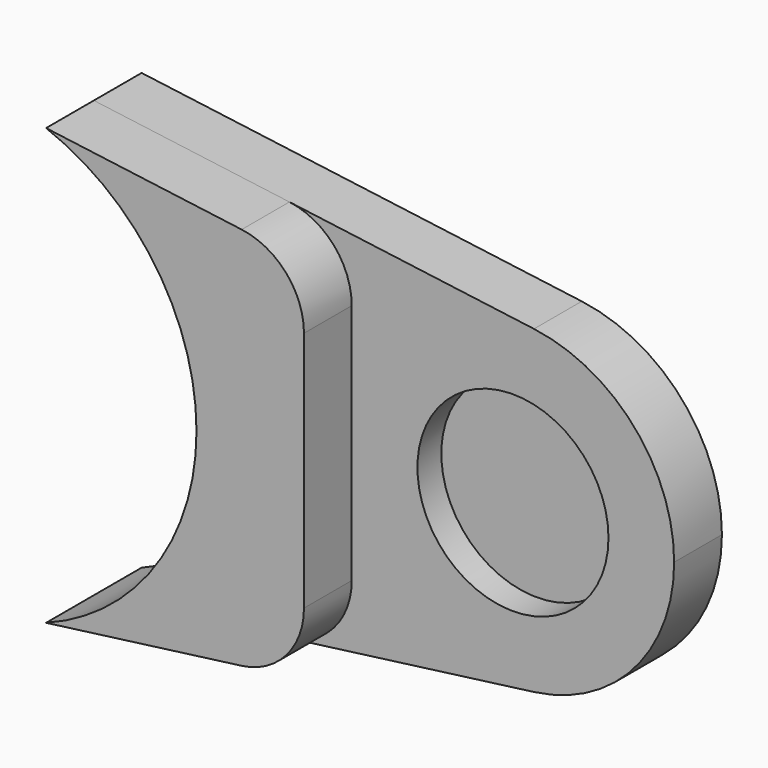
from build123d import *

# Parameters (mm, degrees)
F0_R         = 8
F1_DEPTH     = 10
F2_R         = 1.5
F3_DEPTH     = 22.1
F4_R         = 1.4
F5_DEPTH     = 8
F6_T1_DEPTH  = 25.4217528018
F7_R         = 2
F8_R         = 2
F10_DEPTH    = 2.5
F11_R        = 4
F12_DEPTH    = 6
F14_DEPTH    = 2.5
F15_T1_DEPTH = 9.0773234724
F17_DEPTH    = 25
F18_DEPTH    = 7.25


# Not quite as in the source:
# - a fillet or chamfer that OpenCascade refuses, or shapes differently, is made with other operations: its cross-section is extruded or revolved along the edge and cut away or added


with BuildPart() as f1:
    # F0 (on Front) → F1 (new body)
    with BuildSketch(Plane.XZ):
        with BuildLine():
            ThreePointArc((-5.123475383, -8), (4.5594398703, -8.3343570879), (9.5, 0))
            ThreePointArc((9.5, 0), (2.5991730895, 9.1375215048), (-8.0777472107, 5))
            ThreePointArc((-8.0777472107, 5), (-8.4879541617, 4.2666888975), (-8.8317608663, 3.5))
            ThreePointArc((-8.8317608663, 3.5), (-9.0415515645, -2.9155351664), (-5.123475383, -8))
        make_face()
        Circle(F0_R, mode=Mode.SUBTRACT)
        with BuildLine():
            ThreePointArc((-8.8317608663, 3.5), (-8.4879541617, 4.2666888975), (-8.0777472107, 5))
            Line((-8.0777472107, 5), (-23.5, 5))
            ThreePointArc((-23.5, 5), (-24.7247448714, 4.5811388301), (-25.4364916731, 3.5))
            Line((-25.4364916731, 3.5), (-8.8317608663, 3.5))
        make_face()
        with BuildLine():
            Line((-23.5, -8), (-5.123475383, -8))
            ThreePointArc((-5.123475383, -8), (-9.0415515645, -2.9155351664), (-8.8317608663, 3.5))
            Line((-8.8317608663, 3.5), (-25.4364916731, 3.5))
            ThreePointArc((-25.4364916731, 3.5), (-25.4840593925, 3.252008585), (-25.5, 3))
            Line((-25.5, 3), (-25.5, 0))
            Line((-25.5, 0), (-25.5, -3.5))
            Line((-25.5, -3.5), (-25.5, -6))
            ThreePointArc((-25.5, -6), (-24.9142135624, -7.4142135624), (-23.5, -8))
        make_face()
        with BuildLine():
            ThreePointArc((-25.5, 3), (-25.4840593925, 3.252008585), (-25.4364916731, 3.5))
            Line((-25.4364916731, 3.5), (-25.5, 3.5))
            Line((-25.5, 3.5), (-31.5, 3.5))
            ThreePointArc((-31.5, 3.5), (-32.2071067812, 3.2071067812), (-32.5, 2.5))
            Line((-32.5, 2.5), (-32.5, 1.5))
            Line((-32.5, 1.5), (-32.5, 0))
            Line((-32.5, 0), (-32.5, -1.5))
            Line((-32.5, -1.5), (-32.5, -2.5))
            ThreePointArc((-32.5, -2.5), (-32.2071067812, -3.2071067812), (-31.5, -3.5))
            Line((-31.5, -3.5), (-25.5, -3.5))
            Line((-25.5, -3.5), (-25.5, 0))
            Line((-25.5, 0), (-25.5, 3))
        make_face()
    extrude(amount=F1_DEPTH)

    # F2 (on face) → F3 (cut)
    with BuildSketch(Plane(origin=(-32.5, 0, 0), x_dir=(0, -1, 0), z_dir=(-1, 0, 0))):
        with Locations((5, 0)):
            Circle(F2_R)
    extrude(amount=-F3_DEPTH, mode=Mode.SUBTRACT)

    # F4 (on face) → F5 (cut)
    with BuildSketch(Plane(origin=(0, 0, -8), x_dir=(1, 0, 0), z_dir=(0, 0, -1))):
        with Locations((-12.4, 5)):
            Circle(F4_R)
        with Locations((-19.5, 5)):
            Circle(F4_R)
    extrude(amount=-F5_DEPTH, mode=Mode.SUBTRACT)

    # F6: fillet of radius 2 on 2 edges, made by hand

    # F6_s2 → F6_t1 (cut)
    with BuildSketch(Plane.YZ.offset(-28.4997500063)):
        with BuildLine():
            ThreePointArc((-8.0001, 5.0001), (-9.4143135624, 4.4143135624), (-10.0001, 3.0001))
            Line((-10.0001, 3.0001), (-10.0401, 3.0001))
            ThreePointArc((-10.0401, 3.0001), (-10.04, 4.00005), (-10.04, 5))
            Line((-10.04, 5), (-10, 5.04))
            ThreePointArc((-10, 5.04), (-9.00005, 5.04), (-8.0001, 5.0401))
            Line((-8.0001, 5.0401), (-8.0001, 5.0001))
        make_face()
        with BuildLine():
            ThreePointArc((-1.9999, 5.0001), (-0.5856864376, 4.4143135624), (0.0001, 3.0001))
            Line((0.0001, 3.0001), (0.0401, 3.0001))
            ThreePointArc((0.0401, 3.0001), (0.04, 4.00005), (0.04, 5))
            Line((0.04, 5), (0, 5.04))
            ThreePointArc((0, 5.04), (-0.99995, 5.04), (-1.9999, 5.0401))
            Line((-1.9999, 5.0401), (-1.9999, 5.0001))
        make_face()
    extrude(amount=F6_T1_DEPTH, mode=Mode.SUBTRACT)

    # F7
    f7_edges = [f1.edges().sort_by_distance(p)[0] for p in [
        (-32.5, -10, 0),
        (-32.5, 0, 0),
    ]]
    fillet(f7_edges, radius=F7_R)

    # F8
    f8_edges = [f1.edges().sort_by_distance(p)[0] for p in [
        (-14.311738, -10, -8),
        (-14.311738, 0, -8),
    ]]
    fillet(f8_edges, radius=F8_R)

    # F9 (on Front) → F10 (join)
    with BuildSketch(Plane.XZ):
        with BuildLine():
            ThreePointArc((0.8300844627, 8.6718317984), (6.4467419184, 5.8591147448), (8.7114698505, 0))
            Line((8.7114698505, 0), (14.25, 0))
            ThreePointArc((14.25, 0), (16.5494157481, 5.0749187005), (21.8810517975, 6.6922528143))
            Line((21.8810517975, 6.6922528143), (1.6475767802, 9.3560403352))
            Line((1.6475767802, 9.3560403352), (0.8300844627, 9.4636652405))
            Line((0.8300844627, 9.4636652405), (0.8300844627, 8.6718317984))
        make_face()
        with BuildLine():
            Line((14.25, 0), (8.7114698505, 0))
            ThreePointArc((8.7114698505, 0), (6.4467419184, -5.8591147448), (0.8300844627, -8.6718317984))
            Line((0.8300844627, -8.6718317984), (0.8300844627, -9.4636652405))
            Line((0.8300844627, -9.4636652405), (1.6475767802, -9.3560403352))
            Line((1.6475767802, -9.3560403352), (21.8810517975, -6.6922528143))
            ThreePointArc((21.8810517975, -6.6922528143), (16.5494157481, -5.0749187005), (14.25, 0))
        make_face()
        with BuildLine():
            ThreePointArc((21.8810517975, 6.6922528143), (16.5494157481, 5.0749187005), (14.25, 0))
            Line((14.25, 0), (21, 0))
            Line((21, 0), (21.8810517975, -6.6922528143))
            ThreePointArc((21.8810517975, -6.6922528143), (26.0749187005, -4.4505842519), (27.75, 0))
            ThreePointArc((27.75, 0), (26.0749187005, 4.4505842519), (21.8810517975, 6.6922528143))
        make_face()
        with BuildLine():
            Line((21, 0), (14.25, 0))
            ThreePointArc((14.25, 0), (16.5494157481, -5.0749187005), (21.8810517975, -6.6922528143))
            Line((21.8810517975, -6.6922528143), (21, 0))
        make_face()
        with BuildLine():
            Line((1.6475767802, -9.3560403352), (0.8300844627, -9.4636652405))
            ThreePointArc((0.8300844627, -9.4636652405), (1.2399988261, -9.4187261831), (1.6475767802, -9.3560403352))
        make_face()
        with BuildLine():
            ThreePointArc((1.6475767802, 9.3560403352), (1.2399988261, 9.4187261831), (0.8300844627, 9.4636652405))
            Line((0.8300844627, 9.4636652405), (1.6475767802, 9.3560403352))
        make_face()
    extrude(amount=F10_DEPTH)

    # F11 (on face) → F12 (join)
    with BuildSketch(Plane.XZ.offset(2.5)):
        with Locations((21, 0)):
            Circle(F11_R)
    extrude(amount=F12_DEPTH)

    # F13 (on face) → F14 (join)
    with BuildSketch(Plane.XZ.offset(2.5)):
        with BuildLine():
            Line((14.25, -7.6968998426), (14.25, 0))
            Line((14.25, 0), (14.25, 7.6968998426))
            Line((14.25, 7.6968998426), (1.6475767802, 9.3560403352))
            Line((1.6475767802, 9.3560403352), (1.6475767802, 8.3387943225))
            ThreePointArc((1.6475767802, 8.3387943225), (8.5, 0), (1.6475767802, -8.3387943225))
            Line((1.6475767802, -8.3387943225), (1.6475767802, -9.3560403352))
            Line((1.6475767802, -9.3560403352), (14.25, -7.6968998426))
        make_face()
    extrude(amount=F14_DEPTH)

    # F15: fillet of radius 3 on 2 edges, made by hand

    # F15_s2 → F15_t1 (cut)
    with BuildSketch(Plane.XZ.offset(2.5)):
        with BuildLine():
            ThreePointArc((11.6415785767, 8.0403050378), (13.5055194224, 7.044007899), (14.25, 5.0659704537))
            Line((14.25, 5.0659704537), (14.25, 7.6968998426))
            Line((14.25, 7.6968998426), (11.6415785767, 8.0403050378))
        make_face()
        with BuildLine():
            ThreePointArc((14.25, -5.0659704537), (13.5055194224, -7.044007899), (11.6415785767, -8.0403050378))
            Line((11.6415785767, -8.0403050378), (14.25, -7.6968998426))
            Line((14.25, -7.6968998426), (14.25, -5.0659704537))
        make_face()
    extrude(amount=F15_T1_DEPTH, mode=Mode.SUBTRACT)

    # F16 (on face) → F17 (cut)
    with BuildSketch(Plane.XZ.offset(10)):
        with BuildLine():
            Line((-37.4530367553, -9.75), (0, -9.75))
            ThreePointArc((0, -9.75), (9.75, 0), (0, 9.75))
            Line((0, 9.75), (0, 13.4185552597))
            Line((0, 13.4185552597), (-34.6982963383, 13.4185552597))
            Line((-34.6982963383, 13.4185552597), (-37.4530367553, 13.4185552597))
            Line((-37.4530367553, 13.4185552597), (-37.4530367553, -9.75))
        make_face()
    extrude(amount=-F17_DEPTH, mode=Mode.SUBTRACT)

    # F18 (cut): a face of the model
    f18_faces = [f1.faces().sort_by_distance(p)[0] for p in [
        (21, -8.5, 0),
    ]]
    extrude(f18_faces, amount=-F18_DEPTH, mode=Mode.SUBTRACT)


solid = f1.part
